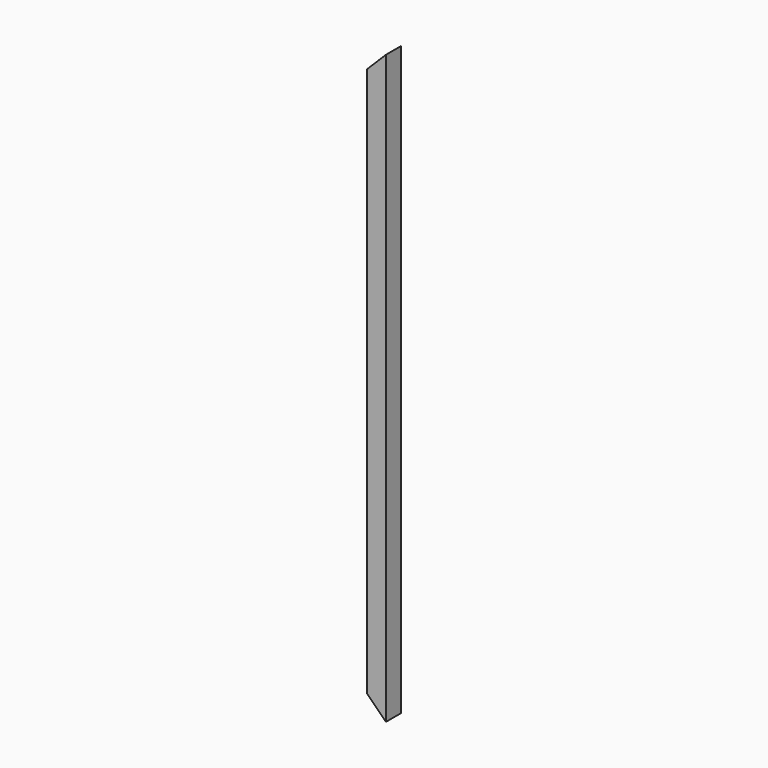
from build123d import *

# Parameters (mm, degrees)
F0_W        = 40
F0_H        = 40
F0_W_2      = 36
F0_H_2      = 36
F1_DEPTH    = 1250
F2_T1_DEPTH = 245.7346390373


# Not quite as in the source:
# - a fillet or chamfer that OpenCascade refuses, or shapes differently, is made with other operations: its cross-section is extruded or revolved along the edge and cut away or added


with BuildPart() as f1:
    # F0 (on Top) → F1 (new body)
    with BuildSketch(Plane.XY):
        with Locations((20, 20)):
            Rectangle(F0_W, F0_H)
        with Locations((20, 20)):
            Rectangle(F0_W_2, F0_H_2, mode=Mode.SUBTRACT)
    extrude(amount=F1_DEPTH)

    # F2: chamfer of 40 on 2 edges, made by hand

    # F2_s2 → F2_t1 (cut)
    with BuildSketch(Plane.XZ.offset(-142.8673195186)):
        Polygon((0, 40), (40, 0), (0, 0), align=None)
        Polygon((0, 1210), (40, 1250), (0, 1250), align=None)
    extrude(amount=F2_T1_DEPTH, mode=Mode.SUBTRACT)


solid = f1.part
